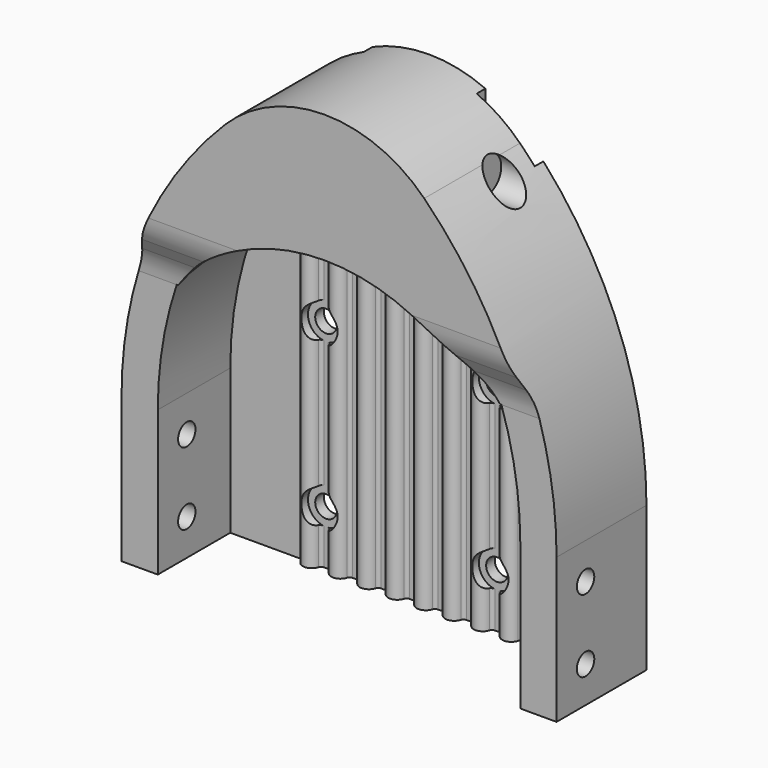
from build123d import *

# Parameters (mm, degrees)
F1_DEPTH       = 3
F3_DEPTH       = 25
F6_R           = 1
F10_R          = 5
F11_DEPTH      = 5
F11_DEPTH_BACK = 25
F12_R          = 5
F13_DEPTH      = 5
F13_DEPTH_BACK = 25
F14_R          = 3
F15_DEPTH      = 25
F16_R          = 5
F17_DEPTH      = 25
F19_DEPTH      = 3
F21_DEPTH      = 5
F23_DEPTH      = 60.0010001
F23_DEPTH_BACK = 60.0010001
F24_R          = 3
F25_DEPTH      = 120.0010001


with BuildPart() as f1:
    # F0 (on Front) → F1 (new body)
    with BuildSketch(Plane.XZ):
        with BuildLine():
            ThreePointArc((0, 130), (-14.8864619161, 127.0344226607), (-27.5, 118.5904867099))
            ThreePointArc((-27.5, 118.5904867099), (-51.5544962217, 82.5226839501), (-60, 40))
            Line((-60, 40), (-60, 0))
            Line((-60, 0), (0, 0))
            Line((0, 0), (60, 0))
            Line((60, 0), (60, 40))
            ThreePointArc((60, 40), (51.5544962217, 82.5226839501), (27.5, 118.5904867099))
            ThreePointArc((27.5, 118.5904867099), (14.8864619161, 127.0344226607), (0, 130))
        make_face()
    extrude(amount=F1_DEPTH)

    # F2 (on face) → F3 (join)
    with BuildSketch(Plane.XZ.offset(3)):
        with BuildLine():
            ThreePointArc((60, 40), (51.5544962217, 82.5226839501), (27.5, 118.5904867099))
            ThreePointArc((27.5, 118.5904867099), (0, 130), (-27.5, 118.5904867099))
            ThreePointArc((-27.5, 118.5904867099), (-51.5544962217, 82.5226839501), (-60, 40))
            Line((-60, 40), (-60, 0))
            Line((-60, 0), (-50, 0))
            Line((-50, 0), (-50, 40))
            ThreePointArc((-50, 40), (-45.21984083, 70.746507549), (-31.3306193747, 98.5904867099))
            ThreePointArc((-31.3306193747, 98.5904867099), (-16.6083160845, 106.784974752), (0, 109.6239332364))
            ThreePointArc((0, 109.6239332364), (16.6083160845, 106.784974752), (31.3306193747, 98.5904867099))
            ThreePointArc((31.3306193747, 98.5904867099), (45.21984083, 70.746507549), (50, 40))
            Line((50, 40), (50, 0))
            Line((50, 0), (60, 0))
            Line((60, 0), (60, 40))
        make_face()
    extrude(amount=F3_DEPTH)

    # F4 (on face) → F5 (join, up to the next surface of F1)
    with BuildSketch(Plane(origin=(0, 0, 0), x_dir=(1, 0, 0), z_dir=(0, 0, -1))):
        with BuildLine():
            Line((25, 3), (30, 3))
            ThreePointArc((30, 3), (27.5, 5.5), (25, 3))
        make_face()
        with BuildLine():
            Line((17.1428571429, 3), (22.1428571429, 3))
            ThreePointArc((22.1428571429, 3), (19.6428571429, 5.5), (17.1428571429, 3))
        make_face()
        with BuildLine():
            Line((9.2857142857, 3), (14.2857142857, 3))
            ThreePointArc((14.2857142857, 3), (11.7857142857, 5.5), (9.2857142857, 3))
        make_face()
        with BuildLine():
            Line((1.4285714286, 3), (6.4285714286, 3))
            ThreePointArc((6.4285714286, 3), (3.9285714286, 5.5), (1.4285714286, 3))
        make_face()
        with BuildLine():
            Line((-6.4285714286, 3), (-1.4285714286, 3))
            ThreePointArc((-1.4285714286, 3), (-3.9285714286, 5.5), (-6.4285714286, 3))
        make_face()
        with BuildLine():
            Line((-14.2857142857, 3), (-9.2857142857, 3))
            ThreePointArc((-9.2857142857, 3), (-11.7857142857, 5.5), (-14.2857142857, 3))
        make_face()
        with BuildLine():
            Line((-22.1428571429, 3), (-17.1428571429, 3))
            ThreePointArc((-17.1428571429, 3), (-19.6428571429, 5.5), (-22.1428571429, 3))
        make_face()
        with BuildLine():
            Line((-30, 3), (-25, 3))
            ThreePointArc((-25, 3), (-27.5, 5.5), (-30, 3))
        make_face()
    extrude(until=Until.NEXT, dir=(0, 0, 1))

    # F6
    f6_edges = [f1.edges().sort_by_distance(p)[0] for p in [
        (25, -3, 51.462602),
        (30, -3, 49.811967),
        (22.142857, -3, 52.226771),
        (14.285714, -3, 53.769838),
        (6.428571, -3, 54.604473),
        (-1.428571, -3, 54.80176),
        (-9.285714, -3, 54.377061),
        (-17.142857, -3, 53.296656),
        (-25, -3, 51.462602),
        (17.142857, -3, 53.296656),
        (9.285714, -3, 54.377061),
        (1.428571, -3, 54.80176),
        (-6.428571, -3, 54.604473),
        (-14.285714, -3, 53.769838),
        (-22.142857, -3, 52.226771),
        (-30, -3, 49.811967),
    ]]
    fillet(f6_edges, radius=F6_R)

    # F10 (on offset) → F11 (cut, two sides)
    with BuildSketch(Plane.YZ.offset(31.337)) as f11_sk:
        with Locations((-10, 114.5469088508)):
            Circle(F10_R)
    extrude(amount=-F11_DEPTH, mode=Mode.SUBTRACT)
    extrude(f11_sk.sketch, amount=F11_DEPTH_BACK, mode=Mode.SUBTRACT)

    # F12 (on offset) → F13 (cut, two sides)
    with BuildSketch(Plane.YZ.offset(-31.337)) as f13_sk:
        with Locations((-10, 114.5469088508)):
            Circle(F12_R)
    extrude(amount=F13_DEPTH, mode=Mode.SUBTRACT)
    extrude(f13_sk.sketch, amount=-F13_DEPTH_BACK, mode=Mode.SUBTRACT)

    # F14 (on face) → F15 (cut)
    with BuildSketch(Plane.XZ.offset(3)):
        with Locations((23.5714285714, 15)):
            Circle(F14_R)
        with Locations((23.5714285714, 60)):
            Circle(F14_R)
        with Locations((-23.5714285714, 15)):
            Circle(F14_R)
        with Locations((-23.5714285714, 60)):
            Circle(F14_R)
    extrude(amount=-F15_DEPTH, mode=Mode.SUBTRACT)

    # F16 (on face) → F17 (cut)
    with BuildSketch(Plane.XZ.offset(3)):
        with Locations((-23.5714285714, 60)):
            Circle(F16_R)
        with Locations((23.5714285714, 60)):
            Circle(F16_R)
        with Locations((23.5714285714, 15)):
            Circle(F16_R)
        with Locations((-23.5714285714, 15)):
            Circle(F16_R)
    extrude(amount=F17_DEPTH, mode=Mode.SUBTRACT)

    # F18 (on face) → F19 (join)
    with BuildSketch(Plane(origin=(0, 0, 0), x_dir=(-1, 0, 0), z_dir=(0, 1, 0))):
        with BuildLine():
            Line((-31.5714285714, 0), (-31.5714285714, 114.2863015176))
            ThreePointArc((-31.5714285714, 114.2863015176), (-52.6501162334, 79.7700838151), (-60, 40))
            Line((-60, 40), (-60, 0))
            Line((-60, 0), (-31.5714285714, 0))
        make_face()
        with BuildLine():
            Line((-15.5714285714, 0), (0, 0))
            Line((0, 0), (15.5714285714, 0))
            Line((15.5714285714, 0), (15.5714285714, 126.7425103309))
            ThreePointArc((15.5714285714, 126.7425103309), (0, 130), (-15.5714285714, 126.7425103309))
            Line((-15.5714285714, 126.7425103309), (-15.5714285714, 0))
        make_face()
        with BuildLine():
            Line((31.5714285714, 114.2863015176), (31.5714285714, 0))
            Line((31.5714285714, 0), (60, 0))
            Line((60, 0), (60, 40))
            ThreePointArc((60, 40), (52.6501162334, 79.7700838151), (31.5714285714, 114.2863015176))
        make_face()
    extrude(amount=F19_DEPTH)

    # F20 (on face) → F21 (join)
    with BuildSketch(Plane.XZ.offset(28)):
        with BuildLine():
            ThreePointArc((27.5, 118.5904867099), (0, 130), (-27.5, 118.5904867099))
            ThreePointArc((-27.5, 118.5904867099), (-44.5249877256, 96.6075224882), (-55.5684147451, 71.0900060985))
            Line((-55.5684147451, 71.0900060985), (-45.109713573, 71.0900060985))
            ThreePointArc((-45.109713573, 71.0900060985), (0, 94.6239332364), (45.109713573, 71.0900060985))
            Line((45.109713573, 71.0900060985), (55.5684147451, 71.0900060985))
            ThreePointArc((55.5684147451, 71.0900060985), (44.5249877256, 96.6075224882), (27.5, 118.5904867099))
        make_face()
    extrude(amount=F21_DEPTH)

    # F22 (on Right) → F23 (cut, two sides)
    with BuildSketch(Plane.YZ) as f23_sk:
        with BuildLine():
            ThreePointArc((-28, 72.0900060985), (-28.4177080594, 75.6052246919), (-29.6475682345, 78.924665267))
            Line((-29.6475682345, 78.924665267), (-31.3524317655, 82.2553469301))
            ThreePointArc((-31.3524317655, 82.2553469301), (-32.5822919406, 85.5747875052), (-33, 89.0900060985))
            Line((-33, 89.0900060985), (-33, 92.9825796194))
            Line((-33, 92.9825796194), (-39.6550593126, 92.9825796194))
            Line((-39.6550593126, 92.9825796194), (-39.6550593126, 71.0900060985))
            Line((-39.6550593126, 71.0900060985), (-28, 71.0900060985))
            Line((-28, 71.0900060985), (-28, 72.0900060985))
        make_face()
    extrude(amount=-F23_DEPTH, mode=Mode.SUBTRACT)
    extrude(f23_sk.sketch, amount=F23_DEPTH_BACK, mode=Mode.SUBTRACT)

    # F24 (on face) → F25 (cut, through all)
    with BuildSketch(Plane(origin=(-60, 0, 0), x_dir=(0, -1, 0), z_dir=(-1, 0, 0))):
        with Locations((18, 10)):
            Circle(F24_R)
        with Locations((18, 30)):
            Circle(F24_R)
    extrude(amount=-F25_DEPTH, mode=Mode.SUBTRACT)


solid = f1.part
